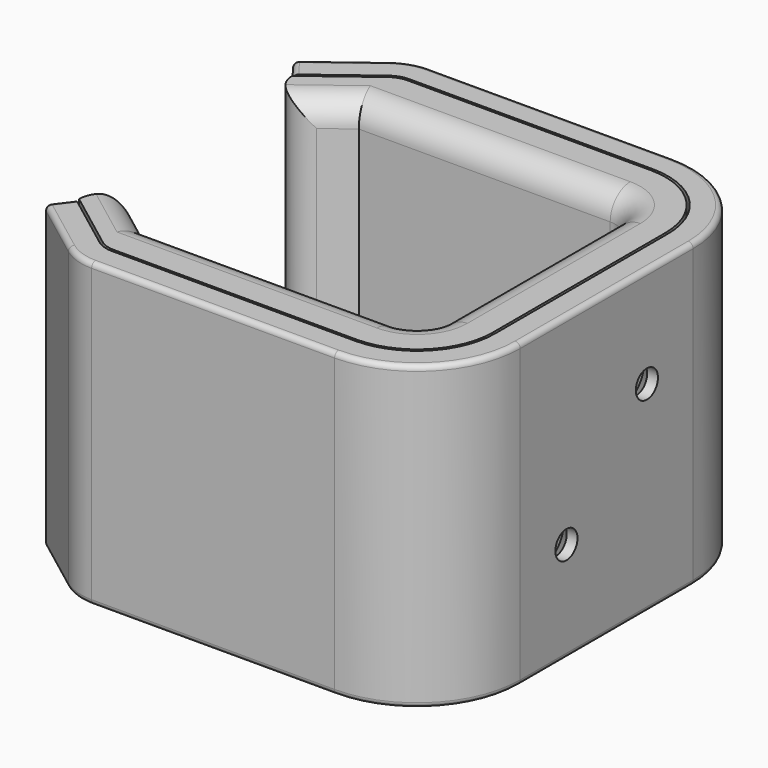
from build123d import *

# Parameters (mm, degrees)
F1_DEPTH       = 60
F3_W           = 48.3226891947
F3_H           = 4.5
F4_DEPTH       = 5
F5_DEPTH       = 60
F6_T1_DEPTH    = 110.2402603275
F6_T3_DEPTH    = 43
F6_T8_DEPTH    = 41.582121483
F6_T13_DEPTH   = 62.5
F6_T18_DEPTH   = 41.582121483
F6_T23_DEPTH   = 41.582121483
F6_T28_DEPTH   = 41.582121483
F6_T33_DEPTH   = 62.5
F6_T36_ANGLE   = 90
F6_T38_ANGLE   = 90
F6_T42_DEPTH   = 62.5
F6_T45_ANGLE   = 90
F6_T49_DEPTH   = 62.5
F6_T52_ANGLE   = 90
F6_T57_DEPTH   = 41.582121483
F6_T61_DEPTH   = 62.5
F6_T68_DEPTH   = 62.5
F6_T72_DEPTH   = 41.582121483
F6_T79_DEPTH   = 62.5
F6_T83_DEPTH   = 41.582121483
F6_T90_DEPTH   = 62.5
F6_T94_DEPTH   = 41.582121483
F8_D           = 5.5
F8_DEPTH       = 12
F8_CSINK_D     = 11.2
F8_CSINK_ANGLE = 90
F8_TIP         = 1.6523667023
F9_W           = 48.3226891947
F9_H           = 5
F10_DEPTH      = 5
F11_W          = 48.3226891947
F11_H          = 5
F12_DEPTH      = 5
F13_R          = 1


# Not quite as in the source:
# - a fillet or chamfer that OpenCascade refuses, or shapes differently, is made with other operations: its cross-section is extruded or revolved along the edge and cut away or added


with BuildPart() as f1:
    # F0 (on Top) → F1 (new body)
    with BuildSketch(Plane.XY):
        with BuildLine():
            ThreePointArc((27.5, -21.5), (26.0355339059, -25.0355339059), (22.5, -26.5))
            Line((22.5, -26.5), (-27.5, -26.5))
            Line((-27.5, -26.5), (-40.7274998724, -16.5))
            Line((-40.7274998724, -16.5), (-40.7274998724, -26.5))
            Line((-40.7274998724, -26.5), (-28.8379849186, -35.4884823803))
            ThreePointArc((-28.8379849186, -35.4884823803), (-27.4129074343, -36.2403803593), (-25.8226891947, -36.5))
            Line((-25.8226891947, -36.5), (22.5, -36.5))
            ThreePointArc((22.5, -36.5), (33.1066017178, -32.1066017178), (37.5, -21.5))
            Line((37.5, -21.5), (37.5, 21.5))
            ThreePointArc((37.5, 21.5), (33.1066017178, 32.1066017178), (22.5, 36.5))
            Line((22.5, 36.5), (-25.8226891947, 36.5))
            ThreePointArc((-25.8226891947, 36.5), (-27.4129074343, 36.2403803593), (-28.8379849186, 35.4884823803))
            Line((-28.8379849186, 35.4884823803), (-40.7274998724, 26.5))
            Line((-40.7274998724, 26.5), (-40.7274998724, 16.5))
            Line((-40.7274998724, 16.5), (-27.5, 26.5))
            Line((-27.5, 26.5), (22.5, 26.5))
            ThreePointArc((22.5, 26.5), (26.0355339059, 25.0355339059), (27.5, 21.5))
            Line((27.5, 21.5), (27.5, -21.5))
        make_face()
    extrude(amount=F1_DEPTH)

    # F3 (on face) → F4 (cut)
    with BuildSketch(Plane(origin=(0, 0, 0), x_dir=(1, 0, 0), z_dir=(0, 0, -1))):
        with Locations((-1.6613445974, 34.25)):
            Rectangle(F3_W, F3_H)
        with Locations((-1.6613445974, -34.25)):
            Rectangle(F3_W, F3_H)
    extrude(amount=-F4_DEPTH, mode=Mode.SUBTRACT)

    # F6: fillet of radius 5 on 16 edges, made by hand

    # F6_s2 → F6_t1 (cut)
    with BuildSketch(Plane.XY.offset(-25.1201301638)):
        with BuildLine():
            ThreePointArc((-32.7122041486, 22.5595696852), (-37.9550008692, 22.0716428673), (-40.7274998724, 26.5480520655))
            Line((-40.7274998724, 26.5480520655), (-40.7274998724, 16.5))
            Line((-40.7274998724, 16.5), (-32.7122041486, 22.5595696852))
        make_face()
        with BuildLine():
            ThreePointArc((-32.7122041486, -22.5595696852), (-37.9550008692, -22.0716428673), (-40.7274998724, -26.5480520655))
            Line((-40.7274998724, -26.5480520655), (-40.7274998724, -16.5))
            Line((-40.7274998724, -16.5), (-32.7122041486, -22.5595696852))
        make_face()
    extrude(amount=F6_T1_DEPTH, mode=Mode.SUBTRACT)

    # F6_s4 → F6_t3 (cut)
    with BuildSketch(Plane.XZ.offset(-21.5)):
        with BuildLine():
            ThreePointArc((27.5, 5), (28.9644660941, 1.4644660941), (32.5, 0))
            Line((32.5, 0), (27.5, 0))
            Line((27.5, 0), (27.5, 5))
        make_face()
        with BuildLine():
            ThreePointArc((27.5, 55), (28.9644660941, 58.5355339059), (32.5, 60))
            Line((32.5, 60), (27.5, 60))
            Line((27.5, 60), (27.5, 55))
        make_face()
    extrude(amount=F6_T3_DEPTH, mode=Mode.SUBTRACT)


with BuildPart() as f5:
    # F2 (on Top) → F5 (new body)
    with BuildSketch(Plane.XY):
        with BuildLine():
            Line((-29.139514491, -35.8873306183), (-41.0291804666, -26.8987340655))
            Line((-41.0291804666, -26.8987340655), (-43.4414170456, -30.0895199697))
            ThreePointArc((-43.4414170456, -30.0895199697), (-43.6342043679, -30.8302084913), (-43.2467797144, -31.4902755905))
            Line((-43.2467797144, -31.4902755905), (-32.1548102148, -39.8758129986))
            ThreePointArc((-32.1548102148, -39.8758129986), (-29.1621474978, -41.4547987545), (-25.8226891947, -42))
            Line((-25.8226891947, -42), (22.5, -42))
            ThreePointArc((22.5, -42), (36.9956890143, -35.9956890143), (43, -21.5))
            Line((43, -21.5), (43, 21.5))
            ThreePointArc((43, 21.5), (36.9956890143, 35.9956890143), (22.5, 42))
            Line((22.5, 42), (-25.8226891947, 42))
            ThreePointArc((-25.8226891947, 42), (-29.1621474978, 41.4547987545), (-32.1548102148, 39.8758129986))
            Line((-32.1548102148, 39.8758129986), (-43.2467797144, 31.4902755905))
            ThreePointArc((-43.2467797144, 31.4902755905), (-43.6342043679, 30.8302084913), (-43.4414170456, 30.0895199697))
            Line((-43.4414170456, 30.0895199697), (-41.0291804666, 26.8987340655))
            Line((-41.0291804666, 26.8987340655), (-29.139514491, 35.8873306183))
            ThreePointArc((-29.139514491, 35.8873306183), (-27.5719292582, 36.7144183952), (-25.8226891947, 37))
            Line((-25.8226891947, 37), (22.5, 37))
            ThreePointArc((22.5, 37), (33.4601551084, 32.4601551084), (38, 21.5))
            Line((38, 21.5), (38, -21.5))
            ThreePointArc((38, -21.5), (33.4601551084, -32.4601551084), (22.5, -37))
            Line((22.5, -37), (-25.8226891947, -37))
            ThreePointArc((-25.8226891947, -37), (-27.5719292582, -36.7144183952), (-29.139514491, -35.8873306183))
        make_face()
    extrude(amount=F5_DEPTH)

    # F8
    with Locations(Plane(origin=(38, 0, 0), x_dir=(0, -1, 0), z_dir=(-1, 0, 0))):
        with Locations((-10, 40), (10, 20)):
            CounterSinkHole(F8_D / 2, F8_CSINK_D / 2, depth=F8_DEPTH, counter_sink_angle=F8_CSINK_ANGLE)
            with Locations((0, 0, -(F8_DEPTH + F8_TIP / 2))):  # 118° drill point
                Cone(0, F8_D / 2, F8_TIP, mode=Mode.SUBTRACT)

    # F9 (on face) → F10 (join)
    with BuildSketch(Plane.XZ.offset(-37)):
        with Locations((-1.6613445974, 2.5)):
            Rectangle(F9_W, F9_H)
    extrude(amount=F10_DEPTH)

    # F11 (on face) → F12 (join)
    with BuildSketch(Plane(origin=(0, -37, 0), x_dir=(-1, 0, 0), z_dir=(0, 1, 0))):
        with Locations((1.6613445974, 2.5)):
            Rectangle(F11_W, F11_H)
    extrude(amount=F12_DEPTH)

    # F13
    f13_edges = [f5.edges().sort_by_distance(p)[0] for p in [
        (-1.661345, 42, 60),
        (-37.700795, 35.683044, 0),
        (-42.235299, -28.494127, 0),
        (-42.235299, -28.494127, 60),
        (-43.634204, -30.830208, 0),
        (-37.700795, -35.683044, 0),
        (-29.162147, -41.454799, 0),
        (-1.661345, -42, 0),
        (36.995689, -35.995689, 0),
        (43, 0, 0),
        (36.995689, 35.995689, 0),
        (-1.661345, 42, 0),
        (-29.162147, 41.454799, 0),
        (-43.634204, 30.830208, 0),
        (-42.235299, 28.494127, 0),
        (-43.634204, -30.830208, 60),
        (-37.700795, -35.683044, 60),
        (-29.162147, -41.454799, 60),
        (-1.661345, -42, 60),
        (36.995689, -35.995689, 60),
        (43, 0, 60),
        (36.995689, 35.995689, 60),
        (-29.162147, 41.454799, 60),
        (-37.700795, 35.683044, 60),
        (-43.634204, 30.830208, 60),
        (-42.235299, 28.494127, 60),
    ]]
    fillet(f13_edges, radius=F13_R)


with BuildPart() as f6_tool6:
    # F6_s7 → F6_t8 (new body)
    with BuildSketch(Plane(origin=(-27.9494555927, -21.1298097617, 0), x_dir=(0, 0, 1), z_dir=(0.7976964761, 0.6030591448, 0))):
        with BuildLine():
            ThreePointArc((60, -42.7230830966), (58.5355339059, -39.1875491907), (55, -37.7230830966))
            Line((55, -37.7230830966), (60, -37.7230830966))
            Line((60, -37.7230830966), (60, -42.7230830966))
        make_face()
    extrude(amount=F6_T8_DEPTH)

    split(bisect_by=Plane.XZ.offset(-26.5), keep=Keep.TOP)


with BuildPart() as f1_1:
    add(f1.part)

    # F6_t5: cut F6_tool6
    add(f6_tool6.part, mode=Mode.SUBTRACT)


with BuildPart() as f6_tool11:
    # F6_s12 → F6_t13 (new body)
    with BuildSketch(Plane.YZ.offset(-40)):
        with BuildLine():
            ThreePointArc((31.5, 60), (27.9644660941, 58.5355339059), (26.5, 55))
            Line((26.5, 55), (26.5, 60))
            Line((26.5, 60), (31.5, 60))
        make_face()
    extrude(amount=F6_T13_DEPTH)

    split(bisect_by=Plane(origin=(-22.7492502304, 30.091570452, 0), x_dir=(0, 0, 1), z_dir=(0.6030591448, -0.7976964761, 0)), keep=Keep.TOP)


with BuildPart() as f1_2:
    add(f1_1.part)

    # F6_t10: cut F6_tool11
    add(f6_tool11.part, mode=Mode.SUBTRACT)


with BuildPart() as f6_tool16:
    # F6_s17 → F6_t18 (new body)
    with BuildSketch(Plane(origin=(5.220456181, -3.9466688576, 0), x_dir=(0, 0, 1), z_dir=(-0.7976964761, 0.6030591448, 0))):
        with BuildLine():
            ThreePointArc((60, -42.7230830966), (58.5355339059, -39.1875491907), (55, -37.7230830966))
            Line((55, -37.7230830966), (60, -37.7230830966))
            Line((60, -37.7230830966), (60, -42.7230830966))
        make_face()
    extrude(amount=F6_T18_DEPTH)

    split(bisect_by=Plane.XZ.offset(26.5), keep=Keep.BOTTOM)


with BuildPart() as f1_3:
    add(f1_2.part)

    # F6_t15: cut F6_tool16
    add(f6_tool16.part, mode=Mode.SUBTRACT)


with BuildPart() as f6_tool21:
    # F6_s22 → F6_t23 (new body)
    with BuildSketch(Plane(origin=(-27.9494555927, -21.1298097617, 0), x_dir=(0, 0, 1), z_dir=(0.7976964761, 0.6030591448, 0))):
        with BuildLine():
            ThreePointArc((0, -42.7230830966), (1.4644660941, -39.1875491907), (5, -37.7230830966))
            Line((5, -37.7230830966), (0, -37.7230830966))
            Line((0, -37.7230830966), (0, -42.7230830966))
        make_face()
    extrude(amount=F6_T23_DEPTH)

    split(bisect_by=Plane.XZ.offset(-26.5), keep=Keep.TOP)


with BuildPart() as f1_4:
    add(f1_3.part)

    # F6_t20: cut F6_tool21
    add(f6_tool21.part, mode=Mode.SUBTRACT)


with BuildPart() as f6_tool26:
    # F6_s27 → F6_t28 (new body)
    with BuildSketch(Plane(origin=(5.220456181, -3.9466688576, 0), x_dir=(0, 0, 1), z_dir=(-0.7976964761, 0.6030591448, 0))):
        with BuildLine():
            ThreePointArc((0, -42.7230830966), (1.4644660941, -39.1875491907), (5, -37.7230830966))
            Line((5, -37.7230830966), (0, -37.7230830966))
            Line((0, -37.7230830966), (0, -42.7230830966))
        make_face()
    extrude(amount=F6_T28_DEPTH)

    split(bisect_by=Plane.XZ.offset(26.5), keep=Keep.BOTTOM)


with BuildPart() as f1_5:
    add(f1_4.part)

    # F6_t25: cut F6_tool26
    add(f6_tool26.part, mode=Mode.SUBTRACT)


with BuildPart() as f6_tool31:
    # F6_s32 → F6_t33 (new body)
    with BuildSketch(Plane.YZ.offset(22.5)):
        with BuildLine():
            ThreePointArc((-26.5, 5), (-27.9644660941, 1.4644660941), (-31.5, 0))
            Line((-31.5, 0), (-26.5, 0))
            Line((-26.5, 0), (-26.5, 5))
        make_face()
    extrude(amount=-F6_T33_DEPTH)

    split(bisect_by=Plane(origin=(-22.7492502304, -30.091570452, 0), x_dir=(0, 0, 1), z_dir=(0.6030591448, 0.7976964761, 0)), keep=Keep.TOP)


with BuildPart() as f1_6:
    add(f1_5.part)

    # F6_t30: cut F6_tool31
    add(f6_tool31.part, mode=Mode.SUBTRACT)

    # F6_s35 → F6_t36 (revolve, cut)
    with BuildSketch(Plane.XZ.offset(21.5)):
        with BuildLine():
            ThreePointArc((27.5, 5), (28.9644660941, 1.4644660941), (32.5, 0))
            Line((32.5, 0), (27.5, 0))
            Line((27.5, 0), (27.5, 5))
        make_face()
    revolve(axis=Axis((22.5, -21.5, 0), (0, 0, -1)), revolution_arc=F6_T36_ANGLE, mode=Mode.SUBTRACT)

    # F6_s37 → F6_t38 (revolve, cut)
    with BuildSketch(Plane.XZ.offset(21.5)):
        with BuildLine():
            ThreePointArc((27.5, 55), (28.9644660941, 58.5355339059), (32.5, 60))
            Line((32.5, 60), (27.5, 60))
            Line((27.5, 60), (27.5, 55))
        make_face()
    revolve(axis=Axis((22.5, -21.5, 60), (0, 0, -1)), revolution_arc=F6_T38_ANGLE, mode=Mode.SUBTRACT)


with BuildPart() as f6_tool40:
    # F6_s41 → F6_t42 (new body)
    with BuildSketch(Plane.YZ.offset(22.5)):
        with BuildLine():
            ThreePointArc((-26.5, 55), (-27.9644660941, 58.5355339059), (-31.5, 60))
            Line((-31.5, 60), (-26.5, 60))
            Line((-26.5, 60), (-26.5, 55))
        make_face()
    extrude(amount=-F6_T42_DEPTH)

    split(bisect_by=Plane(origin=(-22.7492502304, -30.091570452, 0), x_dir=(0, 0, 1), z_dir=(0.6030591448, 0.7976964761, 0)), keep=Keep.TOP)


with BuildPart() as f1_7:
    add(f1_6.part)

    # F6_t39: cut F6_tool40
    add(f6_tool40.part, mode=Mode.SUBTRACT)

    # F6_s44 → F6_t45 (revolve, cut)
    with BuildSketch(Plane.YZ.offset(22.5)):
        with BuildLine():
            ThreePointArc((31.5, 0), (27.9644660941, 1.4644660941), (26.5, 5))
            Line((26.5, 5), (26.5, 0))
            Line((26.5, 0), (31.5, 0))
        make_face()
    revolve(axis=Axis((22.5, 21.5, 0), (0, 0, -1)), revolution_arc=F6_T45_ANGLE, mode=Mode.SUBTRACT)


with BuildPart() as f6_tool47:
    # F6_s48 → F6_t49 (new body)
    with BuildSketch(Plane.YZ.offset(-40)):
        with BuildLine():
            ThreePointArc((31.5, 0), (27.9644660941, 1.4644660941), (26.5, 5))
            Line((26.5, 5), (26.5, 0))
            Line((26.5, 0), (31.5, 0))
        make_face()
    extrude(amount=F6_T49_DEPTH)

    split(bisect_by=Plane(origin=(-22.7492502304, 30.091570452, 0), x_dir=(0, 0, 1), z_dir=(0.6030591448, -0.7976964761, 0)), keep=Keep.TOP)


with BuildPart() as f1_8:
    add(f1_7.part)

    # F6_t46: cut F6_tool47
    add(f6_tool47.part, mode=Mode.SUBTRACT)

    # F6_s51 → F6_t52 (revolve, cut)
    with BuildSketch(Plane.YZ.offset(22.5)):
        with BuildLine():
            ThreePointArc((31.5, 60), (27.9644660941, 58.5355339059), (26.5, 55))
            Line((26.5, 55), (26.5, 60))
            Line((26.5, 60), (31.5, 60))
        make_face()
    revolve(axis=Axis((22.5, 21.5, 60), (0, 0, -1)), revolution_arc=F6_T52_ANGLE, mode=Mode.SUBTRACT)


with BuildPart() as f6_tool55:
    # F6_s56 → F6_t57 (new body)
    with BuildSketch(Plane(origin=(-27.9494555927, -21.1298097617, 0), x_dir=(0, 0, 1), z_dir=(0.7976964761, 0.6030591448, 0))):
        with BuildLine():
            ThreePointArc((60, -42.7230830966), (58.5355339059, -39.1875491907), (55, -37.7230830966))
            Line((55, -37.7230830966), (60, -37.7230830966))
            Line((60, -37.7230830966), (60, -42.7230830966))
        make_face()
    extrude(amount=F6_T57_DEPTH)

    split(bisect_by=Plane.XZ.offset(-26.5), keep=Keep.BOTTOM)


with BuildPart() as f6_tool59:
    # F6_s60 → F6_t61 (new body)
    with BuildSketch(Plane.YZ.offset(-40)):
        with BuildLine():
            ThreePointArc((31.5, 60), (27.9644660941, 58.5355339059), (26.5, 55))
            Line((26.5, 55), (26.5, 60))
            Line((26.5, 60), (31.5, 60))
        make_face()
    extrude(amount=F6_T61_DEPTH)

    split(bisect_by=Plane(origin=(-22.7492502304, 30.091570452, 0), x_dir=(0, 0, 1), z_dir=(-0.6030591448, 0.7976964761, 0)), keep=Keep.TOP)


with BuildPart() as f6_tool55_1:
    add(f6_tool55.part)

    # F6_t63: intersect F6_tool59
    add(f6_tool59.part, mode=Mode.INTERSECT)


with BuildPart() as f1_9:
    add(f1_8.part)

    # F6_t53: cut F6_tool55
    add(f6_tool55_1.part, mode=Mode.SUBTRACT)


with BuildPart() as f6_tool66:
    # F6_s67 → F6_t68 (new body)
    with BuildSketch(Plane.YZ.offset(22.5)):
        with BuildLine():
            ThreePointArc((-26.5, 55), (-27.9644660941, 58.5355339059), (-31.5, 60))
            Line((-31.5, 60), (-26.5, 60))
            Line((-26.5, 60), (-26.5, 55))
        make_face()
    extrude(amount=-F6_T68_DEPTH)

    split(bisect_by=Plane(origin=(-22.7492502304, -30.091570452, 0), x_dir=(0, 0, 1), z_dir=(-0.6030591448, -0.7976964761, 0)), keep=Keep.TOP)


with BuildPart() as f6_tool70:
    # F6_s71 → F6_t72 (new body)
    with BuildSketch(Plane(origin=(5.220456181, -3.9466688576, 0), x_dir=(0, 0, 1), z_dir=(-0.7976964761, 0.6030591448, 0))):
        with BuildLine():
            ThreePointArc((60, -42.7230830966), (58.5355339059, -39.1875491907), (55, -37.7230830966))
            Line((55, -37.7230830966), (60, -37.7230830966))
            Line((60, -37.7230830966), (60, -42.7230830966))
        make_face()
    extrude(amount=F6_T72_DEPTH)

    split(bisect_by=Plane.XZ.offset(26.5), keep=Keep.TOP)


with BuildPart() as f6_tool66_1:
    add(f6_tool66.part)

    # F6_t74: intersect F6_tool70
    add(f6_tool70.part, mode=Mode.INTERSECT)


with BuildPart() as f1_10:
    add(f1_9.part)

    # F6_t64: cut F6_tool66
    add(f6_tool66_1.part, mode=Mode.SUBTRACT)


with BuildPart() as f6_tool77:
    # F6_s78 → F6_t79 (new body)
    with BuildSketch(Plane.YZ.offset(-40)):
        with BuildLine():
            ThreePointArc((31.5, 0), (27.9644660941, 1.4644660941), (26.5, 5))
            Line((26.5, 5), (26.5, 0))
            Line((26.5, 0), (31.5, 0))
        make_face()
    extrude(amount=F6_T79_DEPTH)

    split(bisect_by=Plane(origin=(-22.7492502304, 30.091570452, 0), x_dir=(0, 0, 1), z_dir=(-0.6030591448, 0.7976964761, 0)), keep=Keep.TOP)


with BuildPart() as f6_tool81:
    # F6_s82 → F6_t83 (new body)
    with BuildSketch(Plane(origin=(-27.9494555927, -21.1298097617, 0), x_dir=(0, 0, 1), z_dir=(0.7976964761, 0.6030591448, 0))):
        with BuildLine():
            ThreePointArc((0, -42.7230830966), (1.4644660941, -39.1875491907), (5, -37.7230830966))
            Line((5, -37.7230830966), (0, -37.7230830966))
            Line((0, -37.7230830966), (0, -42.7230830966))
        make_face()
    extrude(amount=F6_T83_DEPTH)

    split(bisect_by=Plane.XZ.offset(-26.5), keep=Keep.BOTTOM)


with BuildPart() as f6_tool77_1:
    add(f6_tool77.part)

    # F6_t85: intersect F6_tool81
    add(f6_tool81.part, mode=Mode.INTERSECT)


with BuildPart() as f1_11:
    add(f1_10.part)

    # F6_t75: cut F6_tool77
    add(f6_tool77_1.part, mode=Mode.SUBTRACT)


with BuildPart() as f6_tool88:
    # F6_s89 → F6_t90 (new body)
    with BuildSketch(Plane.YZ.offset(22.5)):
        with BuildLine():
            ThreePointArc((-26.5, 5), (-27.9644660941, 1.4644660941), (-31.5, 0))
            Line((-31.5, 0), (-26.5, 0))
            Line((-26.5, 0), (-26.5, 5))
        make_face()
    extrude(amount=-F6_T90_DEPTH)

    split(bisect_by=Plane(origin=(-22.7492502304, -30.091570452, 0), x_dir=(0, 0, 1), z_dir=(-0.6030591448, -0.7976964761, 0)), keep=Keep.TOP)


with BuildPart() as f6_tool92:
    # F6_s93 → F6_t94 (new body)
    with BuildSketch(Plane(origin=(5.220456181, -3.9466688576, 0), x_dir=(0, 0, 1), z_dir=(-0.7976964761, 0.6030591448, 0))):
        with BuildLine():
            ThreePointArc((0, -42.7230830966), (1.4644660941, -39.1875491907), (5, -37.7230830966))
            Line((5, -37.7230830966), (0, -37.7230830966))
            Line((0, -37.7230830966), (0, -42.7230830966))
        make_face()
    extrude(amount=F6_T94_DEPTH)

    split(bisect_by=Plane.XZ.offset(26.5), keep=Keep.TOP)


with BuildPart() as f6_tool88_1:
    add(f6_tool88.part)

    # F6_t96: intersect F6_tool92
    add(f6_tool92.part, mode=Mode.INTERSECT)


with BuildPart() as f1_12:
    add(f1_11.part)

    # F6_t86: cut F6_tool88
    add(f6_tool88_1.part, mode=Mode.SUBTRACT)


solid = Compound([f5.part, f1_12.part])
